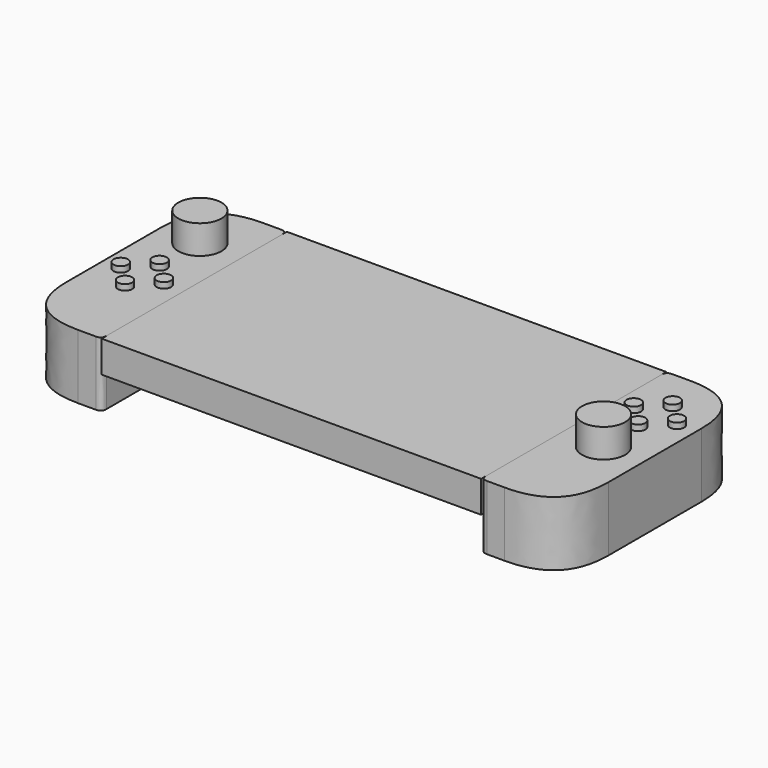
from build123d import *

# Parameters (mm, degrees)
F0_W          = 167.386
F0_H          = 102.108
F1_DEPTH      = 13.97
F2_W          = 35.814
F2_H          = 102.108
F3_DEPTH      = 28.448
F4_W          = 35.814
F4_H          = 102.108
F5_DEPTH      = 28.448
F6_T1_DEPTH   = 155.448
F6_2_T1_DEPTH = 155.448
F7_T1_DEPTH   = 41.148
F7_2_T1_DEPTH = 41.148
F8_R          = 9.525
F9_DEPTH      = 12.7
F10_R         = 3.175
F14_DEPTH     = 2.54
F11_R         = 3.175
F15_DEPTH     = 2.54
F12_R         = 3.175
F13_R         = 3.175
F16_DEPTH     = 2.54
F17_R         = 3.175
F22_DEPTH     = 2.54
F19_R         = 3.175
F23_DEPTH     = 2.54
F20_R         = 3.175
F24_DEPTH     = 2.54
F21_R         = 9.525
F25_DEPTH     = 12.7
F26_R         = 3.175
F27_DEPTH     = 2.54


# Not quite as in the source:
# - a fillet or chamfer that OpenCascade refuses, or shapes differently, is made with other operations: its cross-section is extruded or revolved along the edge and cut away or added


with BuildPart() as f1:
    # F0 (on Top) → F1 (new body)
    with BuildSketch(Plane.XY):
        Rectangle(F0_W, F0_H)
    extrude(amount=F1_DEPTH)


with BuildPart() as f3:
    # F2 (on face) → F3 (new body)
    with BuildSketch(Plane.XY.offset(13.97)):
        with Locations((-101.6, 0)):
            Rectangle(F2_W, F2_H)
    extrude(amount=-F3_DEPTH)

    # F6: fillet of radius 25.4 on 2 edges, made by hand

    # F6_s2 → F6_t1 (cut)
    with BuildSketch(Plane.XY.offset(-77.978)):
        with BuildLine():
            add(Edge.make_bspline(
                [(-94.107, 51.054), (-119.507, 51.054), (-119.507, 25.654)],
                knots=[0, 0, 0, 1, 1, 1], degree=2, weights=[1, 1, 1]))
            Line((-119.507, 25.654), (-119.507, 51.054))
            Line((-119.507, 51.054), (-94.107, 51.054))
        make_face()
        with BuildLine():
            add(Edge.make_bspline(
                [(-119.507, -25.654), (-119.507, -51.054), (-94.107, -51.054)],
                knots=[0, 0, 0, 1, 1, 1], degree=2, weights=[1, 1, 1]))
            Line((-94.107, -51.054), (-119.507, -51.054))
            Line((-119.507, -51.054), (-119.507, -25.654))
        make_face()
    extrude(amount=F6_T1_DEPTH, mode=Mode.SUBTRACT)

    # F7: fillet of radius 2.54 on 2 edges, made by hand

    # F7_s2 → F7_t1 (cut)
    with BuildSketch(Plane.XY.offset(-20.828)):
        with BuildLine():
            add(Edge.make_bspline(
                [(-83.693, 48.514), (-83.693, 51.054), (-86.233, 51.054)],
                knots=[0, 0, 0, 1, 1, 1], degree=2, weights=[1, 1, 1]))
            Line((-86.233, 51.054), (-83.693, 51.054))
            Line((-83.693, 51.054), (-83.693, 48.514))
        make_face()
        with BuildLine():
            add(Edge.make_bspline(
                [(-83.693, -48.514), (-83.693, -51.054), (-86.233, -51.054)],
                knots=[0, 0, 0, 1, 1, 1], degree=2, weights=[1, 1, 1]))
            Line((-86.233, -51.054), (-83.693, -51.054))
            Line((-83.693, -51.054), (-83.693, -48.514))
        make_face()
    extrude(amount=F7_T1_DEPTH, mode=Mode.SUBTRACT)


with BuildPart() as f5:
    # F4 (on face) → F5 (new body)
    with BuildSketch(Plane.XY.offset(13.97)):
        with Locations((101.6, 0)):
            Rectangle(F4_W, F4_H)
    extrude(amount=-F5_DEPTH)

    # F6#2: fillet of radius 25.4 on 2 edges, made by hand

    # F6_2_s2 → F6_2_t1 (cut)
    with BuildSketch(Plane.XY.offset(-77.978)):
        with BuildLine():
            add(Edge.make_bspline(
                [(94.107, 51.054), (119.507, 51.054), (119.507, 25.654)],
                knots=[0, 0, 0, 1, 1, 1], degree=2, weights=[1, 1, 1]))
            Line((119.507, 25.654), (119.507, 51.054))
            Line((119.507, 51.054), (94.107, 51.054))
        make_face()
        with BuildLine():
            add(Edge.make_bspline(
                [(94.107, -51.054), (119.507, -51.054), (119.507, -25.654)],
                knots=[0, 0, 0, 1, 1, 1], degree=2, weights=[1, 1, 1]))
            Line((119.507, -25.654), (119.507, -51.054))
            Line((119.507, -51.054), (94.107, -51.054))
        make_face()
    extrude(amount=F6_2_T1_DEPTH, mode=Mode.SUBTRACT)

    # F7#2: fillet of radius 2.54 on 2 edges, made by hand

    # F7_2_s2 → F7_2_t1 (cut)
    with BuildSketch(Plane.XY.offset(-20.828)):
        with BuildLine():
            add(Edge.make_bspline(
                [(86.233, 51.054), (83.693, 51.054), (83.693, 48.514)],
                knots=[0, 0, 0, 1, 1, 1], degree=2, weights=[1, 1, 1]))
            Line((83.693, 48.514), (83.693, 51.054))
            Line((83.693, 51.054), (86.233, 51.054))
        make_face()
        with BuildLine():
            add(Edge.make_bspline(
                [(83.693, -48.514), (83.693, -51.054), (86.233, -51.054)],
                knots=[0, 0, 0, 1, 1, 1], degree=2, weights=[1, 1, 1]))
            Line((86.233, -51.054), (83.693, -51.054))
            Line((83.693, -51.054), (83.693, -48.514))
        make_face()
    extrude(amount=F7_2_T1_DEPTH, mode=Mode.SUBTRACT)


with BuildPart() as f9:
    # F8 (on face) → F9 (new body)
    with BuildSketch(Plane.XY.offset(13.97)):
        with Locations((-101.727, 25.654)):
            Circle(F8_R)
    extrude(amount=F9_DEPTH)


with BuildPart() as f14:
    # F10 (on face) → F14 (new body)
    with BuildSketch(Plane.XY.offset(13.97)):
        with Locations((-101.727, 3.429)):
            Circle(F10_R)
    extrude(amount=F14_DEPTH)


with BuildPart() as f15:
    # F11 (on face) → F15 (new body)
    with BuildSketch(Plane.XY.offset(13.97)):
        with Locations((-101.727, -15.621)):
            Circle(F11_R)
    extrude(amount=F15_DEPTH)


with BuildPart() as f15b:
    # F12 (on face) → F15, piece 2 (new body)
    with BuildSketch(Plane.XY.offset(13.97)):
        with Locations((-92.202, -6.096)):
            Circle(F12_R)
    extrude(amount=F15_DEPTH)


with BuildPart() as f16:
    # F13 (on face) → F16 (new body)
    with BuildSketch(Plane.XY.offset(13.97)):
        with Locations((-111.252, -6.096)):
            Circle(F13_R)
    extrude(amount=F16_DEPTH)


with BuildPart() as f22:
    # F17 (on face) → F22 (new body)
    with BuildSketch(Plane.XY.offset(13.97)):
        with Locations((101.727, 32.004)):
            Circle(F17_R)
    extrude(amount=F22_DEPTH)


with BuildPart() as f23:
    # F19 (on face) → F23 (new body)
    with BuildSketch(Plane.XY.offset(13.97)):
        with Locations((92.202, 22.479)):
            Circle(F19_R)
    extrude(amount=F23_DEPTH)


with BuildPart() as f24:
    # F20 (on face) → F24 (new body)
    with BuildSketch(Plane.XY.offset(13.97)):
        with Locations((101.727, 12.954)):
            Circle(F20_R)
    extrude(amount=F24_DEPTH)


with BuildPart() as f25:
    # F21 (on face) → F25 (new body)
    with BuildSketch(Plane.XY.offset(13.97)):
        with Locations((101.727, -6.096)):
            Circle(F21_R)
    extrude(amount=F25_DEPTH)


with BuildPart() as f27:
    # F26 (on face) → F27 (new body)
    with BuildSketch(Plane.XY.offset(13.97)):
        with Locations((111.252, 22.479)):
            Circle(F26_R)
    extrude(amount=F27_DEPTH)


solid = Compound([f1.part, f3.part, f5.part, f9.part, f14.part, f15.part, f15b.part, f16.part, f22.part, f23.part, f24.part, f25.part, f27.part])
